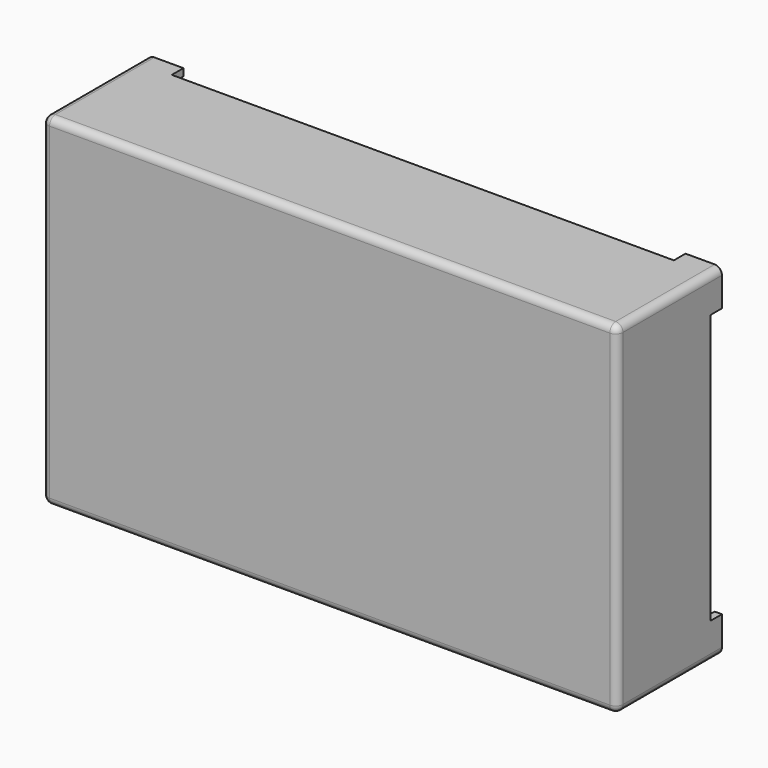
from build123d import *

# Parameters (mm, degrees)
F0_W         = 79
F0_H         = 47
F0_W_2       = 77
F0_H_2       = 45
F1_DEPTH     = 17
F2_W         = 79
F2_H         = 47
F3_DEPTH     = 1
F4_W         = 2
F4_H         = 37
F5_DEPTH     = 79.001
F6_W         = 69
F6_H         = 2
F7_DEPTH     = 47.001
F8_R         = 1
F9_T1_DEPTH  = 19.5
F9_S5_W      = 1
F9_S5_H      = 1
F9_T6_DEPTH  = 1
F9_S11_W     = 1
F9_S11_H     = 1
F9_T12_DEPTH = 1
F9_S17_W     = 1
F9_S17_H     = 1
F9_T18_DEPTH = 1
F9_S23_W     = 1
F9_S23_H     = 1
F9_T24_DEPTH = 1


# Not quite as in the source:
# - a fillet or chamfer that OpenCascade refuses, or shapes differently, is made with other operations: its cross-section is extruded or revolved along the edge and cut away or added


with BuildPart() as f1:
    # F0 (on Front) → F1 (new body)
    with BuildSketch(Plane.XZ):
        with Locations((38.5, 22.5)):
            Rectangle(F0_W, F0_H)
        with Locations((38.5, 22.5)):
            Rectangle(F0_W_2, F0_H_2, mode=Mode.SUBTRACT)
    extrude(amount=F1_DEPTH)

    # F2 (on face) → F3 (join)
    with BuildSketch(Plane.XZ.offset(17)):
        with Locations((38.5, 22.5)):
            Rectangle(F2_W, F2_H)
    extrude(amount=F3_DEPTH)

    # F4 (on face) → F5 (cut, through all)
    with BuildSketch(Plane(origin=(-1, 0, 0), x_dir=(0, -1, 0), z_dir=(-1, 0, 0))):
        with Locations((1, 22.5)):
            Rectangle(F4_W, F4_H)
    extrude(amount=-F5_DEPTH, mode=Mode.SUBTRACT)

    # F6 (on face) → F7 (cut, through all)
    with BuildSketch(Plane(origin=(0, 0, -1), x_dir=(1, 0, 0), z_dir=(0, 0, -1))):
        with Locations((38.5, 1)):
            Rectangle(F6_W, F6_H)
    extrude(amount=-F7_DEPTH, mode=Mode.SUBTRACT)

    # F8
    f8_edges = [f1.edges().sort_by_distance(p)[0] for p in [
        (38.5, -18, 46),
        (-1, -18, 22.5),
        (38.5, -18, -1),
        (78, -18, 22.5),
    ]]
    fillet(f8_edges, radius=F8_R)

    # F9: fillet of radius 1 on 4 edges, made by hand

    # F9_s2 → F9_t1 (cut)
    with BuildSketch(Plane.XZ.offset(-2.5)):
        with BuildLine():
            ThreePointArc((-1, 45), (-0.7071067812, 45.7071067812), (0, 46))
            Line((0, 46), (-1, 46))
            Line((-1, 46), (-1, 45))
        make_face()
        with BuildLine():
            ThreePointArc((-1, 0), (-0.7071067812, -0.7071067812), (0, -1))
            Line((0, -1), (-1, -1))
            Line((-1, -1), (-1, 0))
        make_face()
        with BuildLine():
            ThreePointArc((77, -1), (77.7071067812, -0.7071067812), (78, 0))
            Line((78, 0), (78, -1))
            Line((78, -1), (77, -1))
        make_face()
        with BuildLine():
            ThreePointArc((77, 46), (77.7071067812, 45.7071067812), (78, 45))
            Line((78, 45), (78, 46))
            Line((78, 46), (77, 46))
        make_face()
    extrude(amount=F9_T1_DEPTH, mode=Mode.SUBTRACT)


with BuildPart() as f9_tool4:
    # F9_s5 → F9_t6 (new body)
    with BuildSketch(Plane.XY.offset(45)):
        with Locations((77.5, -17.5)):
            Rectangle(F9_S5_W, F9_S5_H)
    extrude(amount=F9_T6_DEPTH)

    # F9_s7 → F9_t8 (revolve, cut)
    with BuildSketch(Plane(origin=(77, -17, 45), x_dir=(-0.7071067812, 0.7071067812, 0), z_dir=(0.7071067812, 0.7071067812, 0))):
        with BuildLine():
            ThreePointArc((0, -1), (1, 0), (0, 1))
            Line((0, 1), (0, -1))
        make_face()
    revolve(axis=Axis((77, -17, 45), (0, 0, 1)), mode=Mode.SUBTRACT)


with BuildPart() as f1_1:
    add(f1.part)

    # F9_t3: cut F9_tool4
    add(f9_tool4.part, mode=Mode.SUBTRACT)


with BuildPart() as f9_tool10:
    # F9_s11 → F9_t12 (new body)
    with BuildSketch(Plane.XY):
        with Locations((77.5, -17.5)):
            Rectangle(F9_S11_W, F9_S11_H)
    extrude(amount=-F9_T12_DEPTH)

    # F9_s13 → F9_t14 (revolve, cut)
    with BuildSketch(Plane(origin=(77, -17, 0), x_dir=(-0.7071067812, 0.7071067812, 0), z_dir=(-0.7071067812, -0.7071067812, 0))):
        with BuildLine():
            ThreePointArc((0, -1), (1, 0), (0, 1))
            Line((0, 1), (0, -1))
        make_face()
    revolve(axis=Axis((77, -17, 0), (0, 0, -1)), mode=Mode.SUBTRACT)


with BuildPart() as f1_2:
    add(f1_1.part)

    # F9_t9: cut F9_tool10
    add(f9_tool10.part, mode=Mode.SUBTRACT)


with BuildPart() as f9_tool16:
    # F9_s17 → F9_t18 (new body)
    with BuildSketch(Plane.YZ):
        with Locations((-17.5, -0.5)):
            Rectangle(F9_S17_W, F9_S17_H)
    extrude(amount=-F9_T18_DEPTH)

    # F9_s19 → F9_t20 (revolve, cut)
    with BuildSketch(Plane(origin=(0, -17, 0), x_dir=(0, 0.7071067812, 0.7071067812), z_dir=(0, -0.7071067812, 0.7071067812))):
        with BuildLine():
            ThreePointArc((0, -1), (1, 0), (0, 1))
            Line((0, 1), (0, -1))
        make_face()
    revolve(axis=Axis((0, -17, 0), (-1, 0, 0)), mode=Mode.SUBTRACT)


with BuildPart() as f1_3:
    add(f1_2.part)

    # F9_t15: cut F9_tool16
    add(f9_tool16.part, mode=Mode.SUBTRACT)


with BuildPart() as f9_tool22:
    # F9_s23 → F9_t24 (new body)
    with BuildSketch(Plane.YZ):
        with Locations((-17.5, 45.5)):
            Rectangle(F9_S23_W, F9_S23_H)
    extrude(amount=-F9_T24_DEPTH)

    # F9_s25 → F9_t26 (revolve, cut)
    with BuildSketch(Plane(origin=(0, -17, 45), x_dir=(0, 0.7071067812, -0.7071067812), z_dir=(0, 0.7071067812, 0.7071067812))):
        with BuildLine():
            ThreePointArc((0, -1), (1, 0), (0, 1))
            Line((0, 1), (0, -1))
        make_face()
    revolve(axis=Axis((0, -17, 45), (-1, 0, 0)), mode=Mode.SUBTRACT)


with BuildPart() as f1_4:
    add(f1_3.part)

    # F9_t21: cut F9_tool22
    add(f9_tool22.part, mode=Mode.SUBTRACT)


solid = f1_4.part
